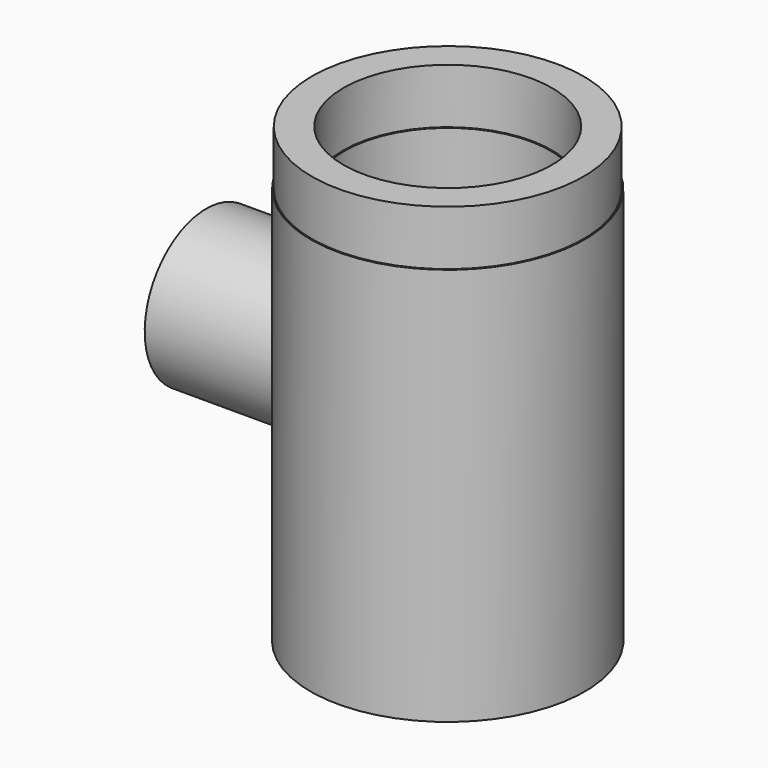
from build123d import *

# Parameters (mm, degrees)
F0_W     = 25
F0_H     = 1
F0_W_2   = 76
F0_W_3   = 75
F3_R     = 55
F4_DEPTH = 176
F5_R     = 75
F6_DEPTH = 1200


# Not quite as in the source:
# - a feature names something its author has since deleted; it is built from what else it names


with BuildPart() as f1:
    # F0 (on Front) → F1 (revolve)
    with BuildSketch(Plane.XZ):
        Polygon((-100, -55), (-75, -55), (-75, 126), (-76, 126), (-76, 166), (-99, 166), (-99, 126), (-100, 126), align=None)
        with Locations((-87.5, -55.5)):
            Rectangle(F0_W, F0_H)
        Polygon((-76, -164), (-75, -164), (-75, -56), (-100, -56), (-100, -164), (-99, -164), (-99, -124), (-76, -124), align=None)
    revolve(axis=Axis((0, 0, -35.4669196472), (0, 0, -1)))

    # F0 (on Front) → F2 (revolve)
    with BuildSketch(Plane.XZ):
        with Locations((-138, -55.5)):
            Rectangle(F0_W_2, F0_H)
        with Locations((-87.5, -55.5)):
            Rectangle(F0_W, F0_H)
        with Locations((-37.5, -55.5)):
            Rectangle(F0_W_3, F0_H)
    revolve(axis=Axis((-175, 0, 0), (-1, 0, 0)))

    # F3 (on face) → F4 (cut, through all)
    with BuildSketch(Plane(origin=(-176, 0, 0), x_dir=(0, -1, 0), z_dir=(-1, 0, 0))):
        Circle(F3_R)
    extrude(amount=-F4_DEPTH, mode=Mode.SUBTRACT)

    # F5 (on face) → F6 (cut)
    with BuildSketch(Plane.XY.offset(166)):
        Circle(F5_R)
    extrude(amount=-F6_DEPTH, mode=Mode.SUBTRACT)


solid = f1.part
